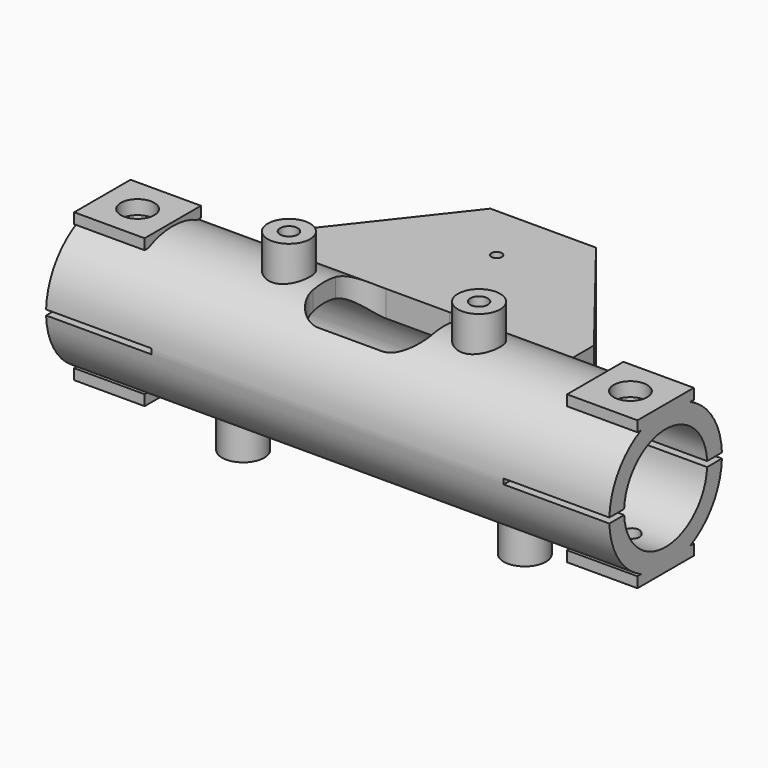
from build123d import *

# Parameters (mm, degrees)
F0_R            = 10
F0_R_2          = 7.375
F1_DEPTH        = 40
F3_DEPTH        = 8
F4_W            = 44
F4_H            = 5.8466901832
F5_W            = 44
F5_H            = 5.8466901832
F6_DEPTH        = 10
F7_W            = 10
F7_H            = 10.75
F8_DEPTH        = 18
F10_W           = 10
F10_H           = 10
F11_DEPTH       = 1.5
F13_W           = 10
F13_H           = 10
F14_DEPTH       = 1.5
F15_R           = 3
F16_DEPTH       = 5.7
F18_D           = 2.5
F18_CBORE_D     = 4.75
F18_CBORE_DEPTH = 2
F20_D           = 2.5
F20_DEPTH       = 8
F20_TIP         = 0.7510757738
F21_R           = 3
F22_DEPTH       = 5.75
F24_D           = 2.5
F24_DEPTH       = 8
F24_TIP         = 0.7510757738
F25_R           = 7.375
F26_DEPTH       = 80.0010001
F27_R           = 2
F28_DEPTH       = 1.5
F29_W           = 17
F29_H           = 12
F30_DEPTH       = 25
F31_R           = 4
F33_DEPTH       = 15
F35_DEPTH       = 15
F36_R           = 0.75
F37_DEPTH       = 25


with BuildPart() as f1:
    # F0 (on Right) → F1 (new body, symmetric)
    with BuildSketch(Plane.YZ):
        Circle(F0_R)
        Circle(F0_R_2, mode=Mode.SUBTRACT)
    extrude(amount=F1_DEPTH, both=True)

    # F2 (on Top) → F3 (join, symmetric)
    with BuildSketch(Plane.XY):
        Polygon((-7.5, 28.2654112475), (-22, 9.7654112475), (22, 9.7654112475), (7.5, 28.2654112475), align=None)
    extrude(amount=F3_DEPTH, both=True)

    # F4 (on face) + F5 (on face) → F6 (join)
    with BuildSketch(Plane.XZ.offset(-9.7654112475)):
        with Locations((0, 5.0766549084)):
            Rectangle(F4_W, F4_H)
    with BuildSketch(Plane.XZ.offset(-9.7654112475)):
        with Locations((0, -5.0766549084)):
            Rectangle(F5_W, F5_H)
    extrude(amount=F6_DEPTH)

    # F7 (on face) → F8 (cut)
    with BuildSketch(Plane(origin=(0, 28.2654112475, 0), x_dir=(-1, 0, 0), z_dir=(0, 1, 0))):
        Rectangle(F7_W, F7_H)
    extrude(amount=-F8_DEPTH, mode=Mode.SUBTRACT)

    # F10 (on offset) → F11 (join)
    with BuildSketch(Plane.XY.offset(9)):
        with Locations((-35, 0)):
            Rectangle(F10_W, F10_H)
        with Locations((35, 0)):
            Rectangle(F10_W, F10_H)
    extrude(amount=F11_DEPTH)

    # F13 (on offset) → F14 (join)
    with BuildSketch(Plane.XY.offset(-9)):
        with Locations((-35, 0)):
            Rectangle(F13_W, F13_H)
        with Locations((35, 0)):
            Rectangle(F13_W, F13_H)
    extrude(amount=-F14_DEPTH)

    # F15 (on offset) → F16 (join)
    with BuildSketch(Plane.XY.offset(9)):
        with Locations((-13.5, 0)):
            Circle(F15_R)
        with Locations((13.5, 0)):
            Circle(F15_R)
    extrude(amount=F16_DEPTH)

    # F18 (through all)
    with Locations(Plane.XY.offset(10.5)):
        with Locations((-35, 0), (35, 0)):
            CounterBoreHole(F18_D / 2, F18_CBORE_D / 2, F18_CBORE_DEPTH)

    # F20
    with Locations(Plane.XY.offset(14.7)):
        with Locations((-13.5, 0), (13.5, 0)):
            Hole(F20_D / 2, depth=F20_DEPTH)
            with Locations((0, 0, -(F20_DEPTH + F20_TIP / 2))):  # 118° drill point
                Cone(0, F20_D / 2, F20_TIP, mode=Mode.SUBTRACT)

    # F21 (on offset) → F22 (join)
    with BuildSketch(Plane.XY.offset(-9)):
        with Locations((-20, 0)):
            Circle(F21_R)
        with Locations((20, 0)):
            Circle(F21_R)
    extrude(amount=-F22_DEPTH)

    # F24
    with Locations(Plane(origin=(0, 0, -14.75), x_dir=(1, 0, 0), z_dir=(0, 0, -1))):
        with Locations((-20, 0), (20, 0)):
            Hole(F24_D / 2, depth=F24_DEPTH)
            with Locations((0, 0, -(F24_DEPTH + F24_TIP / 2))):  # 118° drill point
                Cone(0, F24_D / 2, F24_TIP, mode=Mode.SUBTRACT)

    # F25 (on face) → F26 (cut, through all)
    with BuildSketch(Plane.YZ.offset(40)):
        Circle(F25_R)
    extrude(amount=-F26_DEPTH, mode=Mode.SUBTRACT)

    # F27 (on face) → F28 (cut)
    with BuildSketch(Plane(origin=(0, 0, -10.5), x_dir=(1, 0, 0), z_dir=(0, 0, -1))):
        with Locations((35, 0)):
            Circle(F27_R)
        with Locations((-35, 0)):
            Circle(F27_R)
    extrude(amount=-F28_DEPTH, mode=Mode.SUBTRACT)

    # F29 (on Top) → F30 (cut)
    with BuildSketch(Plane.XY):
        Rectangle(F29_W, F29_H)
    extrude(amount=F30_DEPTH, mode=Mode.SUBTRACT)

    # F31
    f31_edges = [f1.edges().sort_by_distance(p)[0] for p in [
        (8.5, 6, 6.144215),
        (-8.5, 6, 6.144215),
        (-8.5, -6, 6.144215),
        (8.5, -6, 6.144215),
    ]]
    fillet(f31_edges, radius=F31_R)

    # F32 (on face) → F33 (cut)
    with BuildSketch(Plane.YZ.offset(40)):
        with BuildLine():
            Line((-9.9929662763, 0.375), (-12.5, 0.375))
            Line((-12.5, 0.375), (-12.5, -0.375))
            Line((-12.5, -0.375), (-9.9929662763, -0.375))
            ThreePointArc((-9.9929662763, -0.375), (-10, 0), (-9.9929662763, 0.375))
        make_face()
        with BuildLine():
            Line((-7.3654599313, 0.375), (-9.9929662763, 0.375))
            ThreePointArc((-9.9929662763, 0.375), (-10, 0), (-9.9929662763, -0.375))
            Line((-9.9929662763, -0.375), (-7.3654599313, -0.375))
            ThreePointArc((-7.3654599313, -0.375), (-7.375, 0), (-7.3654599313, 0.375))
        make_face()
        with BuildLine():
            Line((9.9929662763, 0.375), (7.3654599313, 0.375))
            ThreePointArc((7.3654599313, 0.375), (7.3726145971, 0.1875606655), (7.375, 0))
            ThreePointArc((7.375, 0), (7.3726145971, -0.1875606655), (7.3654599313, -0.375))
            Line((7.3654599313, -0.375), (9.9929662763, -0.375))
            ThreePointArc((9.9929662763, -0.375), (9.9982414145, -0.1875329793), (10, 0))
            ThreePointArc((10, 0), (9.9982414145, 0.1875329793), (9.9929662763, 0.375))
        make_face()
    extrude(amount=-F33_DEPTH, mode=Mode.SUBTRACT)

    # F34 (on face) → F35 (cut)
    with BuildSketch(Plane(origin=(-40, 0, 0), x_dir=(0, -1, 0), z_dir=(-1, 0, 0))):
        with BuildLine():
            Line((-7.3654599313, 0.375), (-9.9929662763, 0.375))
            ThreePointArc((-9.9929662763, 0.375), (-9.9982414145, 0.1875329793), (-10, 0))
            ThreePointArc((-10, 0), (-9.9982414145, -0.1875329793), (-9.9929662763, -0.375))
            Line((-9.9929662763, -0.375), (-7.3654599313, -0.375))
            ThreePointArc((-7.3654599313, -0.375), (-7.375, 0), (-7.3654599313, 0.375))
        make_face()
        with BuildLine():
            Line((9.9929662763, 0.375), (7.3654599313, 0.375))
            ThreePointArc((7.3654599313, 0.375), (7.3726145971, 0.1875606655), (7.375, 0))
            ThreePointArc((7.375, 0), (7.3726145971, -0.1875606655), (7.3654599313, -0.375))
            Line((7.3654599313, -0.375), (9.9929662763, -0.375))
            ThreePointArc((9.9929662763, -0.375), (10, 0), (9.9929662763, 0.375))
        make_face()
        with BuildLine():
            Line((13.2813919336, 0.375), (9.9929662763, 0.375))
            ThreePointArc((9.9929662763, 0.375), (10, 0), (9.9929662763, -0.375))
            Line((9.9929662763, -0.375), (13.2813919336, -0.375))
            Line((13.2813919336, -0.375), (13.2813919336, 0.375))
        make_face()
    extrude(amount=-F35_DEPTH, mode=Mode.SUBTRACT)

    # F36 (on face) → F37 (cut)
    with BuildSketch(Plane.XY.offset(8)):
        with Locations((0, 19.9929662763)):
            Circle(F36_R)
    extrude(amount=-F37_DEPTH, mode=Mode.SUBTRACT)


solid = f1.part
